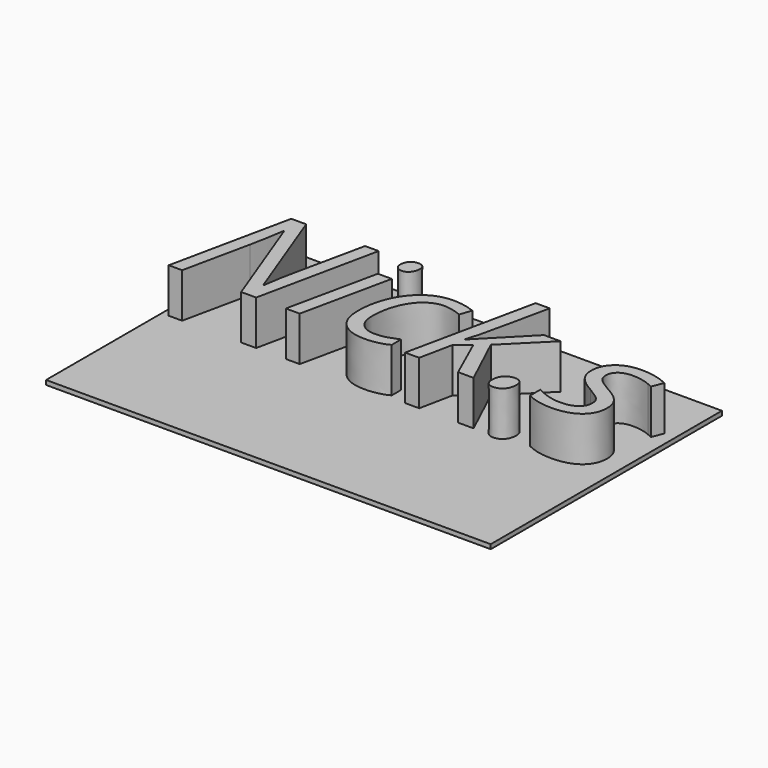
from build123d import *

# Parameters (mm, degrees)
F0_W         = 127
F0_H         = 76.2
F1_DEPTH     = 1.27
F2_TEXT_SIZE = 48.4703917944
F3_DEPTH     = 12.7
F5_DEPTH     = 1.27


# Not quite as in the source:
# - Text() gives the source's letters only with a copy of the font that has no kerning and outlines rounded to 1/6400 em; it was checked with that copy


with BuildPart() as f1:
    # F0 (on Top) → F1 (new body)
    with BuildSketch(Plane.XY):
        with Locations((-12.9801502228, 13.6524992943)):
            Rectangle(F0_W, F0_H)
    extrude(amount=F1_DEPTH)

    # F2 (on face) → F3 (join)
    with BuildSketch(Plane.XY.offset(1.27)):
        with Locations((-76.4801502228, 16.8538172023)):
            Text('Nick.s', F2_TEXT_SIZE, font='Open Sans', font_style=FontStyle.ITALIC, text_align=(TextAlign.LEFT, TextAlign.BOTTOM))
    extrude(amount=F3_DEPTH)

    # F4 (on face) → F5 (join)
    with BuildSketch(Plane.XY.offset(1.27)):
        with BuildLine():
            Line((4.4529250666, 51.7524992943), (50.5198497772, 51.7524992943))
            Line((50.5198497772, 51.7524992943), (50.5198497772, 58.1024992943))
            Line((50.5198497772, 58.1024992943), (-76.4801502228, 58.1024992943))
            Line((-76.4801502228, 58.1024992943), (-76.4801502228, 51.7524992943))
            Line((-76.4801502228, 51.7524992943), (-33.4735959299, 51.7524992943))
            add(Edge.make_bspline(
                [(-33.4735959299, 51.7524992943), (-33.5576748248, 51.6737867201), (-34.3942178476, 50.7452239648), (-34.3942178476, 49.4198616892)],
                knots=[6.9454086014, 6.9454086014, 6.9454086014, 7.0544527696, 8.0972776321, 8.0972776321, 8.0972776321], degree=2))
            add(Edge.make_bspline(
                [(-34.3942178476, 49.4198616892), (-34.3942178476, 48.35199837), (-33.1673110553, 47.1932530661), (-31.1754808925, 47.1932530661), (-29.5926196604, 48.995745761), (-29.5926196604, 51.2288498638), (-29.990746157, 51.7524992943)],
                knots=[0, 0, 0, 1, 2, 3.104, 4.208, 4.9965747418, 4.9965747418, 4.9965747418], degree=2))
            Line((-29.990746157, 51.7524992943), (0.4282573736, 51.7524992943))
            Line((0.4282573736, 51.7524992943), (-6.9705789901, 16.8538172023))
            Line((-6.9705789901, 16.8538172023), (-2.949051171, 16.8538172023))
            Line((-2.949051171, 16.8538172023), (-1.0026620005, 26.3434110958))
            Line((-1.0026620005, 26.3434110958), (2.5947498905, 29.2592081022))
            Line((2.5947498905, 29.2592081022), (8.1536979494, 16.8538172023))
            Line((8.1536979494, 16.8538172023), (12.5766212007, 16.8538172023))
            Line((12.5766212007, 16.8538172023), (5.6014288815, 31.7433156817))
            Line((5.6014288815, 31.7433156817), (16.6966045032, 42.793050311))
            Line((16.6966045032, 42.793050311), (11.9404473084, 42.793050311))
            Line((11.9404473084, 42.793050311), (-0.5103845838, 30.0847194624))
            Line((-0.5103845838, 30.0847194624), (-0.6012665684, 30.0847194624))
            add(Edge.make_bspline(
                [(-0.6012665684, 30.0847194624), (0.4590232521, 33.1368394458), (2.9964785864, 44.9569745187), (4.4529250666, 51.7524992943)],
                knots=[0, 0, 0, 1, 1.876997221, 1.876997221, 1.876997221], degree=2))
        make_face()
    extrude(amount=-F5_DEPTH)


solid = f1.part
